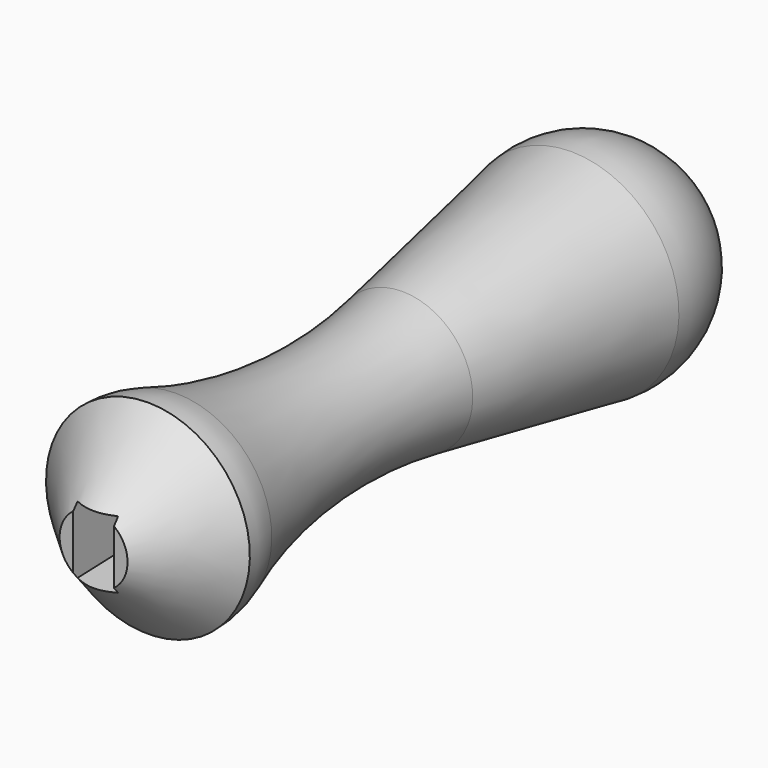
from build123d import *

# Parameters (mm, degrees)
F0_W = 6
F0_H = 10
F2_W = 3
F2_H = 3


# Not quite as in the source:
# - ends of sketch curves that miss each other by under 0.0002 mm in the source are joined


with BuildPart() as f3:
    # F0 (on Front) → F3 section 0
    with BuildSketch(Plane.XZ):
        Rectangle(F0_W, F0_H)
    # F2 (on offset) → F3 section 1
    with BuildSketch(Plane.XZ.offset(-65)):
        Rectangle(F2_W, F2_H)
    loft()


with BuildPart() as f5:
    # F4 (on Right) → F5 (revolve)
    with BuildSketch(Plane.YZ):
        with BuildLine():
            Line((10, 15), (0, 5))
            Line((0, 5), (0, 0))
            Line((0, 0), (106, 0))
            ThreePointArc((106, 0), (100.5324895422, 12.0443623345), (87.8666669945, 15.8571400412))
            Line((87.8666669945, 15.8571400412), (56.800088, 10.359742))
            ThreePointArc((56.800088, 10.359742), (35.7475326189, 9.4526994667), (15.1884568347, 14.0740865517))
            ThreePointArc((15.1884568347, 14.0740865517), (12.6352134757, 14.7667074847), (10, 15))
        make_face()
    revolve(axis=Axis((0, 53, 0), (0, 1, 0)))

    # F6: cut F3
    add(f3.part, mode=Mode.SUBTRACT)


solid = f5.part
